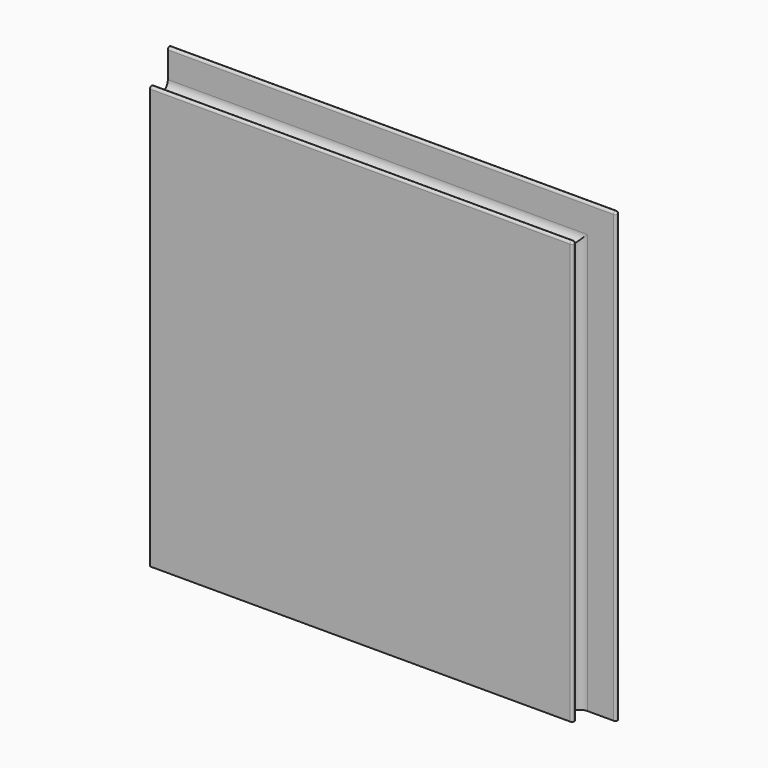
from build123d import *

# Parameters (mm, degrees)
F0_W     = 300
F0_H     = 300
F1_DEPTH = 9
F3_DEPTH = 300.001
F4_R     = 1.49999
F5_R     = 5.99999
F7_DEPTH = 300.001
F8_R     = 5.99999
F9_R     = 1.49999


# Not quite as in the source:
# - a fillet or chamfer is up to 0.001 mm smaller than in the source, because OpenCascade refuses the exact size


with BuildPart() as f1:
    # F0 (on Front) → F1 (new body, symmetric)
    with BuildSketch(Plane.XZ):
        with Locations((-3.7248600274, -5.7776198197)):
            Rectangle(F0_W, F0_H)
    extrude(amount=F1_DEPTH, both=True)

    # F2 (on face) → F3 (cut, through all)
    with BuildSketch(Plane.YZ.offset(146.2751399726)):
        Polygon((6, 144.2223801803), (-9, 144.2223801803), (-9, 127.2223801803), (-6, 127.2223801803), (-6, 119.2223801803), (6, 119.2223801803), align=None)
    extrude(amount=-F3_DEPTH, mode=Mode.SUBTRACT)

    # F4 (radius 1.5 in the source; OpenCascade refuses exactly that, so slightly less here)
    f4_edges = [f1.edges().sort_by_distance(p)[0] for p in [
        (-3.72486, 6, 144.22238),
        (-3.72486, 9, 144.22238),
        (-3.72486, -9, 127.22238),
        (-3.72486, -6, 127.22238),
    ]]
    fillet(f4_edges, radius=F4_R)

    # F5 (radius 6 in the source; OpenCascade refuses exactly that, so slightly less here)
    f5_edges = [f1.edges().sort_by_distance(p)[0] for p in [
        (-3.72486, 6, 119.22238),
        (-3.72486, -6, 119.22238),
    ]]
    fillet(f5_edges, radius=F5_R)

    # F6 (on face) → F7 (cut, through all)
    with BuildSketch(Plane(origin=(0, 0, -155.7776198197), x_dir=(1, 0, 0), z_dir=(0, 0, -1))):
        Polygon((146.2751399726, -6), (146.2751399726, 9), (129.2751399726, 9), (129.2751399726, 6), (121.2751399726, 6), (121.2751399726, -6), align=None)
    extrude(amount=-F7_DEPTH, mode=Mode.SUBTRACT)

    # F8 (radius 6 in the source; OpenCascade refuses exactly that, so slightly less here)
    f8_edges = [f1.edges().sort_by_distance(p)[0] for p in [
        (121.27514, 6, -15.277625),
        (121.27514, -6, -15.277625),
    ]]
    fillet(f8_edges, radius=F8_R)

    # F9 (radius 1.5 in the source; OpenCascade refuses exactly that, so slightly less here)
    f9_edges = [f1.edges().sort_by_distance(p)[0] for p in [
        (129.27514, -6, -15.027615),
        (146.27514, 9, -6.527615),
    ]]
    fillet(f9_edges, radius=F9_R)


solid = f1.part
